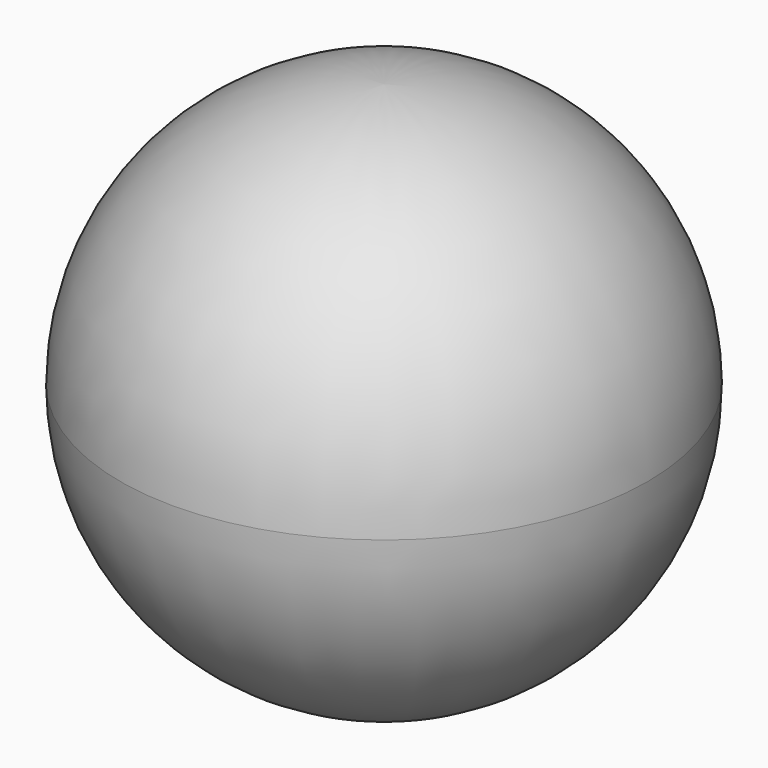
from build123d import *

# Parameters (mm, degrees)
F0_R     = 6.35
F1_DEPTH = 12.7
F2_R     = 6.34999


# Not quite as in the source:
# - a fillet or chamfer is up to 0.001 mm smaller than in the source, because OpenCascade refuses the exact size


with BuildPart() as f1:
    # F0 (on Top) → F1 (new body)
    with BuildSketch(Plane.XY):
        Circle(F0_R)
    extrude(amount=F1_DEPTH)

    # F2 (radius 6.35 in the source; OpenCascade refuses exactly that, so slightly less here)
    f2_edges = [f1.edges().sort_by_distance(p)[0] for p in [
        (-6.35, 0, 12.7),
        (-6.35, 0, 0),
    ]]
    fillet(f2_edges, radius=F2_R)


solid = f1.part
